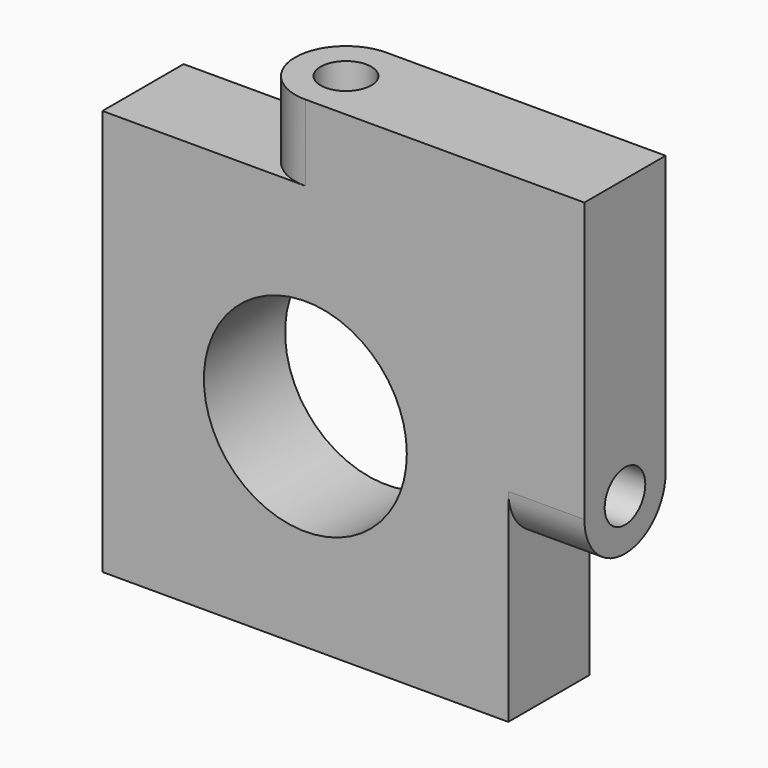
from build123d import *

# Parameters (mm, degrees)
F0_W         = 101.6
F0_H         = 101.6
F1_DEPTH     = 25.4
F2_R         = 6.35
F3_DEPTH     = 19.05
F4_R         = 6.35
F5_DEPTH     = 19.05
F6_R         = 25.4
F7_DEPTH     = 25.4
F8_TEXT_SIZE = 13.2291666667
F9_DEPTH     = 1.905


# Not quite as in the source:
# - Text() gives the source's letters only with a copy of the font that has no kerning and outlines rounded to 1/6400 em; it was checked with that copy


with BuildPart() as f1:
    # F0 (on Front) → F1 (new body)
    with BuildSketch(Plane.XZ):
        with Locations((50.8, 50.8)):
            Rectangle(F0_W, F0_H)
    extrude(amount=F1_DEPTH)

    # F2 (on face) → F3 (join)
    with BuildSketch(Plane.XY.offset(101.6)):
        with BuildLine():
            Line((101.6, 0), (50.8, 0))
            ThreePointArc((50.8, 0), (38.1, -12.7), (50.8, -25.4))
            Line((50.8, -25.4), (101.6, -25.4))
            Line((101.6, -25.4), (101.6, 0))
        make_face()
        with Locations((50.8, -12.7)):
            Circle(F2_R, mode=Mode.SUBTRACT)
    extrude(amount=F3_DEPTH)

    # F4 (on face) → F5 (join)
    with BuildSketch(Plane.YZ.offset(101.6)):
        with BuildLine():
            Line((-25.4, 120.65), (-25.4, 50.8))
            ThreePointArc((-25.4, 50.8), (-12.7, 38.1), (0, 50.8))
            Line((0, 50.8), (0, 120.65))
            Line((0, 120.65), (-25.4, 120.65))
        make_face()
        with Locations((-12.7, 50.8)):
            Circle(F4_R, mode=Mode.SUBTRACT)
    extrude(amount=F5_DEPTH)

    # F6 (on face) → F7 (cut)
    with BuildSketch(Plane.XZ.offset(25.4)):
        with Locations((50.8, 50.8)):
            Circle(F6_R)
    extrude(amount=-F7_DEPTH, mode=Mode.SUBTRACT)

    # F8 (on face) → F9 (join)
    with BuildSketch(Plane(origin=(0, 0, 0), x_dir=(-1, 0, 0), z_dir=(0, 1, 0))):
        with Locations((-111.125, 101.6)):
            Text('politalks', F8_TEXT_SIZE, font='Open Sans', font_style=FontStyle.BOLD, text_align=(TextAlign.LEFT, TextAlign.BOTTOM))
    extrude(amount=F9_DEPTH)


solid = f1.part
